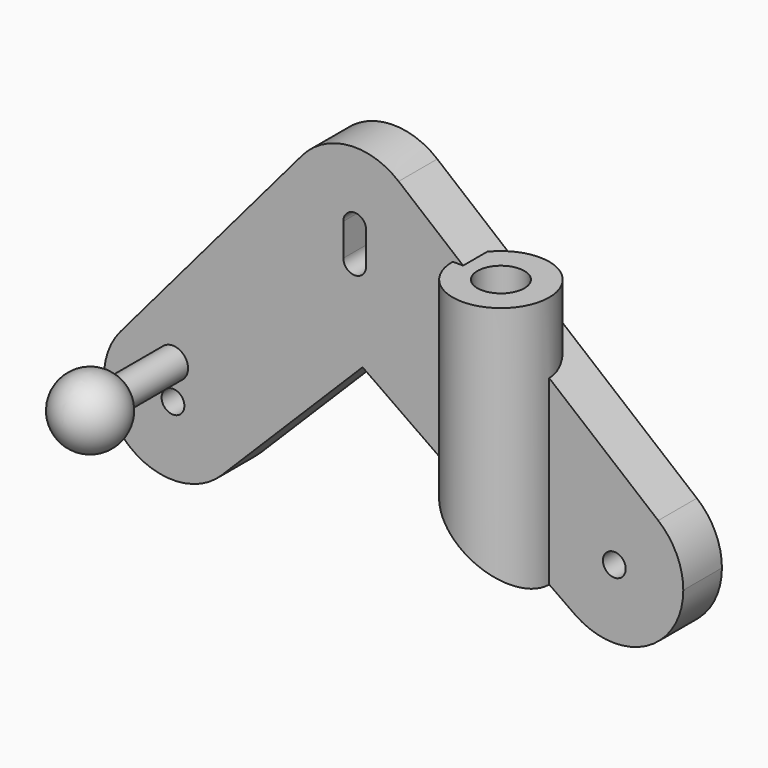
from build123d import *

# Parameters (mm, degrees)
F0_R     = 1.65
F1_DEPTH = 7
F4_R     = 7
F4_R_2   = 3.4
F5_REACH = 60.8499898732
F6_DEPTH = 41.051


with BuildPart() as f1:
    # F0 (on Front) → F1 (new body)
    with BuildSketch(Plane.XZ):
        with BuildLine():
            ThreePointArc((-19.2789321881, -38.1210678119), (-17.1112046749, -34.8768343237), (-16.35, -31.05))
            ThreePointArc((-16.35, -31.05), (-22.9036546106, -21.6626306424), (-33.9745406914, -24.5795765791))
            ThreePointArc((-33.9745406914, -24.5795765791), (-33.1263986939, -38.4039391309), (-19.2789321881, -38.1210678119))
        make_face()
        with Locations((-26.35, -31.05)):
            Circle(F0_R, mode=Mode.SUBTRACT)
        with BuildLine():
            ThreePointArc((-33.9745406914, -24.5795765791), (-22.9036546106, -21.6626306424), (-16.35, -31.05))
            ThreePointArc((-16.35, -31.05), (-17.1112046749, -34.8768343237), (-19.2789321881, -38.1210678119))
            Line((-19.2789321881, -38.1210678119), (1.1377374189, -17.7043982048))
            Line((1.1377374189, -17.7043982048), (-5.7357643635, -12.8915204429))
            ThreePointArc((-5.7357643635, -12.8915204429), (-9.3541818752, -8.2354322855), (-9.7199537036, -2.35))
            ThreePointArc((-9.7199537036, -2.35), (-9.7292260116, 2.3113115789), (-7.6245406914, 6.4704234209))
            Line((-7.6245406914, 6.4704234209), (-33.9745406914, -24.5795765791))
        make_face()
        with BuildLine():
            ThreePointArc((6.3642987803, 7.7133456447), (-0.8850233512, 9.9607596933), (-7.6245406914, 6.4704234209))
            ThreePointArc((-7.6245406914, 6.4704234209), (-9.7292260116, 2.3113115789), (-9.7199537036, -2.35))
            ThreePointArc((-9.7199537036, -2.35), (0, 5.3), (9.7199537036, -2.35))
            ThreePointArc((9.7199537036, -2.35), (9.9297416139, -1.1833137716), (10, 0))
            ThreePointArc((10, 0), (9.0455234178, 4.2636259332), (6.3642987803, 7.7133456447))
        make_face()
        with BuildLine():
            Line((-5.7357643635, -12.8915204429), (1.1377374189, -17.7043982048))
            Line((1.1377374189, -17.7043982048), (7.0710678119, -11.7710678119))
            ThreePointArc((7.0710678119, -11.7710678119), (0.8715574275, -14.6619469809), (-5.7357643635, -12.8915204429))
        make_face()
        with BuildLine():
            Line((7.0710678119, -11.7710678119), (1.1377374189, -17.7043982048))
            Line((1.1377374189, -17.7043982048), (31.8959356141, -39.2415204429))
            ThreePointArc((31.8959356141, -39.2415204429), (29.6730596921, -24.9952460987), (43.995998758, -23.3366543553))
            Line((43.995998758, -23.3366543553), (6.3642987803, 7.7133456447))
            ThreePointArc((6.3642987803, 7.7133456447), (9.0455234178, 4.2636259332), (10, 0))
            ThreePointArc((10, 0), (9.9297416139, -1.1833137716), (9.7199537036, -2.35))
            ThreePointArc((9.7199537036, -2.35), (9.9297416139, -3.5166862284), (10, -4.7))
            ThreePointArc((10, -4.7), (9.2387953251, -8.5268343237), (7.0710678119, -11.7710678119))
        make_face()
        with BuildLine():
            ThreePointArc((43.995998758, -23.3366543553), (29.6730596921, -24.9952460987), (31.8959356141, -39.2415204429))
            ThreePointArc((31.8959356141, -39.2415204429), (42.24918611, -39.9201083318), (47.6316999777, -31.05))
            ThreePointArc((47.6316999777, -31.05), (46.6772233954, -26.7863740668), (43.995998758, -23.3366543553))
        make_face()
        with Locations((37.6316999777, -31.05)):
            Circle(F0_R, mode=Mode.SUBTRACT)
        with BuildLine():
            ThreePointArc((9.7199537036, -2.35), (0, 5.3), (-9.7199537036, -2.35))
            ThreePointArc((-9.7199537036, -2.35), (0, -10), (9.7199537036, -2.35))
        make_face()
        with BuildLine():
            ThreePointArc((-1.65, 0), (0, 1.65), (1.65, 0))
            Line((1.65, 0), (1.65, -4.7))
            ThreePointArc((1.65, -4.7), (0, -6.35), (-1.65, -4.7))
            Line((-1.65, -4.7), (-1.65, 0))
        make_face(mode=Mode.SUBTRACT)
        with BuildLine():
            ThreePointArc((9.7199537036, -2.35), (0, -10), (-9.7199537036, -2.35))
            ThreePointArc((-9.7199537036, -2.35), (-9.3541818752, -8.2354322855), (-5.7357643635, -12.8915204429))
            ThreePointArc((-5.7357643635, -12.8915204429), (0.8715574275, -14.6619469809), (7.0710678119, -11.7710678119))
            ThreePointArc((7.0710678119, -11.7710678119), (9.2387953251, -8.5268343237), (10, -4.7))
            ThreePointArc((10, -4.7), (9.9297416139, -3.5166862284), (9.7199537036, -2.35))
        make_face()
    extrude(amount=F1_DEPTH)

    f5_end = Plane(origin=(16.5168365165, -3.5, -28.4729593239), x_dir=(-0.8191520443, 0, 0.5735764364), z_dir=(-0.5735764364, 0, -0.8191520443))
    # F4 (on Top) → F5 (join, up to a plane its end follows)
    with BuildSketch(Plane.XY):
        with Locations((21.1943648756, -7)):
            Circle(F4_R)
        with Locations((21.1943648756, -7)):
            Circle(F4_R_2, mode=Mode.SUBTRACT)
    f5_long = extrude(amount=-F5_REACH, mode=Mode.PRIVATE)
    add(split(f5_long, bisect_by=f5_end, keep=Keep.BOTTOM, mode=Mode.PRIVATE))

    # F4 (on Top) → F6 (cut, through all)
    with BuildSketch(Plane.XY):
        with Locations((21.1943648756, -7)):
            Circle(F4_R_2)
    extrude(amount=-F6_DEPTH, mode=Mode.SUBTRACT)


with BuildPart() as f3:
    # F2 (on Right) → F3 (revolve)
    with BuildSketch(Plane.YZ):
        with BuildLine():
            Line((-39.9649430722, -1.9130847832), (-50.4749542081, -1.9130847832))
            ThreePointArc((-50.4749542081, -1.9130847832), (-56.0941143788, 0.7577439102), (-59.9649430722, -4.1130847832))
            Line((-59.9649430722, -4.1130847832), (-39.9649430722, -4.1130847832))
            Line((-39.9649430722, -4.1130847832), (-39.9649430722, -1.9130847832))
        make_face()
    revolve(axis=Axis((0, -49.9649430722, -4.1130847832), (0, 1, 0)))


solid = Compound([f1.part, f3.part])
